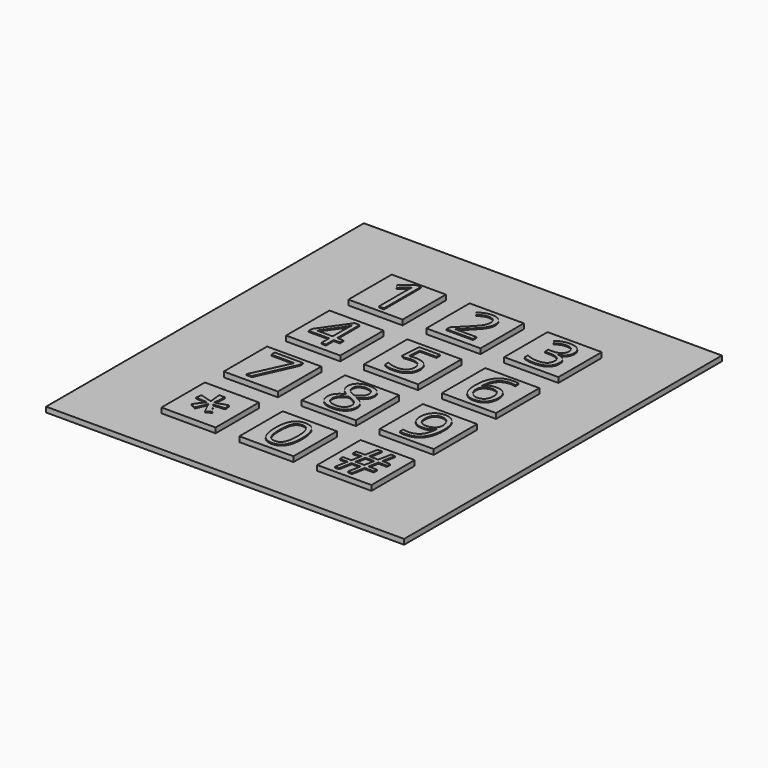
from build123d import *

# Parameters (mm, degrees)
F0_W          = 69.4
F0_H          = 77
F1_DEPTH      = 1
F2_W          = 10.5
F2_H          = 10.5
F3_DEPTH      = 1
F4_TEXT_SIZE  = 12.5769603377
F5_DEPTH      = 0.2
F6_TEXT_SIZE  = 10.9555691274
F7_DEPTH      = 0.2
F8_TEXT_SIZE  = 11.2838111818
F9_DEPTH      = 0.2
F10_TEXT_SIZE = 11.3837614966
F11_DEPTH     = 0.2
F12_TEXT_SIZE = 11.2749830199
F13_DEPTH     = 0.2
F14_TEXT_SIZE = 11.5817846058
F15_DEPTH     = 0.2
F16_TEXT_SIZE = 11.4701903491
F17_DEPTH     = 0.2
F18_TEXT_SIZE = 12.1953906071
F19_DEPTH     = 0.2
F20_TEXT_SIZE = 11.7383821547
F21_DEPTH     = 0.2
F22_TEXT_SIZE = 12.2029864643
F23_DEPTH     = 0.2
F24_TEXT_SIZE = 11.2225185148
F25_DEPTH     = 0.2
F26_TEXT_SIZE = 11.7384957977
F27_DEPTH     = 0.2


# Not quite as in the source:
# - Text() gives the source's letters only with a copy of the font that has no kerning and outlines rounded to 1/6400 em; it was checked with that copy


with BuildPart() as f1:
    # F0 (on Top) → F1 (new body)
    with BuildSketch(Plane.XY):
        with Locations((0.4417933524, 4.7462261665)):
            Rectangle(F0_W, F0_H)
    extrude(amount=F1_DEPTH)


with BuildPart() as f3:
    # F2 (on face) → F3 (new body)
    with BuildSketch(Plane.XY.offset(1)):
        with Locations((-14.0082066476, 25.9962261665)):
            Rectangle(F2_W, F2_H)
    extrude(amount=F3_DEPTH)

    # F4 (on face) → F5 (join)
    with BuildSketch(Plane.XY.offset(2)):
        with Locations((-17.4194090068, 21.5824004263)):
            Text('1', F4_TEXT_SIZE, font='Open Sans', text_align=(TextAlign.LEFT, TextAlign.BOTTOM))
    extrude(amount=F5_DEPTH)


with BuildPart() as f3b:
    # F2 (on face) → F3, piece 2 (new body)
    with BuildSketch(Plane.XY.offset(1)):
        with Locations((-14.0082066476, 10.8962261665)):
            Rectangle(F2_W, F2_H)
    extrude(amount=F3_DEPTH)

    # F10 (on face) → F11 (join)
    with BuildSketch(Plane.XY.offset(2)):
        with Locations((-17.547939904, 6.8340590224)):
            Text('4', F10_TEXT_SIZE, font='Open Sans', text_align=(TextAlign.LEFT, TextAlign.BOTTOM))
    extrude(amount=F11_DEPTH)


with BuildPart() as f3c:
    # F2 (on face) → F3, piece 3 (new body)
    with BuildSketch(Plane.XY.offset(1)):
        with Locations((-14.0082066476, -4.2037738335)):
            Rectangle(F2_W, F2_H)
    extrude(amount=F3_DEPTH)

    # F16 (on face) → F17 (join)
    with BuildSketch(Plane.XY.offset(2)):
        with Locations((-17.3947949011, -8.2585370513)):
            Text('7', F16_TEXT_SIZE, font='Open Sans', text_align=(TextAlign.LEFT, TextAlign.BOTTOM))
    extrude(amount=F17_DEPTH)


with BuildPart() as f3d:
    # F2 (on face) → F3, piece 4 (new body)
    with BuildSketch(Plane.XY.offset(1)):
        with Locations((-14.0082066476, -19.3037738335)):
            Rectangle(F2_W, F2_H)
    extrude(amount=F3_DEPTH)

    # F22 (on face) → F23 (join)
    with BuildSketch(Plane.XY.offset(2)):
        with Locations((-17.4761302769, -25.5072303116)):
            Text('*', F22_TEXT_SIZE, font='Open Sans', text_align=(TextAlign.LEFT, TextAlign.BOTTOM))
    extrude(amount=F23_DEPTH)


with BuildPart() as f3e:
    # F2 (on face) → F3, piece 5 (new body)
    with BuildSketch(Plane.XY.offset(1)):
        with Locations((1.0917933524, 25.9962261665)):
            Rectangle(F2_W, F2_H)
    extrude(amount=F3_DEPTH)

    # F6 (on face) → F7 (join)
    with BuildSketch(Plane.XY.offset(2)):
        with Locations((-1.9074119627, 22.1503581852)):
            Text('2', F6_TEXT_SIZE, font='Open Sans', text_align=(TextAlign.LEFT, TextAlign.BOTTOM))
    extrude(amount=F7_DEPTH)


with BuildPart() as f3f:
    # F2 (on face) → F3, piece 6 (new body)
    with BuildSketch(Plane.XY.offset(1)):
        with Locations((1.0917933524, 10.8962261665)):
            Rectangle(F2_W, F2_H)
    extrude(amount=F3_DEPTH)

    # F12 (on face) → F13 (join)
    with BuildSketch(Plane.XY.offset(2)):
        with Locations((-2.1198638715, 6.924258545)):
            Text('5', F12_TEXT_SIZE, font='Open Sans', text_align=(TextAlign.LEFT, TextAlign.BOTTOM))
    extrude(amount=F13_DEPTH)


with BuildPart() as f3g:
    # F2 (on face) → F3, piece 7 (new body)
    with BuildSketch(Plane.XY.offset(1)):
        with Locations((1.0917933524, -4.2037738335)):
            Rectangle(F2_W, F2_H)
    extrude(amount=F3_DEPTH)

    # F18 (on face) → F19 (join)
    with BuildSketch(Plane.XY.offset(2)):
        with Locations((-2.3180681746, -8.5064787418)):
            Text('8', F18_TEXT_SIZE, font='Open Sans', text_align=(TextAlign.LEFT, TextAlign.BOTTOM))
    extrude(amount=F19_DEPTH)


with BuildPart() as f3h:
    # F2 (on face) → F3, piece 8 (new body)
    with BuildSketch(Plane.XY.offset(1)):
        with Locations((1.0917933524, -19.3037738335)):
            Rectangle(F2_W, F2_H)
    extrude(amount=F3_DEPTH)

    # F24 (on face) → F25 (join)
    with BuildSketch(Plane.XY.offset(2)):
        with Locations((-1.9701938145, -23.3600642532)):
            Text('0', F24_TEXT_SIZE, font='Open Sans', text_align=(TextAlign.LEFT, TextAlign.BOTTOM))
    extrude(amount=F25_DEPTH)


with BuildPart() as f3i:
    # F2 (on face) → F3, piece 9 (new body)
    with BuildSketch(Plane.XY.offset(1)):
        with Locations((16.1917933524, 25.9962261665)):
            Rectangle(F2_W, F2_H)
    extrude(amount=F3_DEPTH)

    # F8 (on face) → F9 (join)
    with BuildSketch(Plane.XY.offset(2)):
        with Locations((13.1029766053, 21.9483301044)):
            Text('3', F8_TEXT_SIZE, font='Open Sans', text_align=(TextAlign.LEFT, TextAlign.BOTTOM))
    extrude(amount=F9_DEPTH)


with BuildPart() as f3j:
    # F2 (on face) → F3, piece 10 (new body)
    with BuildSketch(Plane.XY.offset(1)):
        with Locations((16.1917933524, 10.8962261665)):
            Rectangle(F2_W, F2_H)
    extrude(amount=F3_DEPTH)

    # F14 (on face) → F15 (join)
    with BuildSketch(Plane.XY.offset(2)):
        with Locations((12.8183374181, 6.8138097413)):
            Text('6', F14_TEXT_SIZE, font='Open Sans', text_align=(TextAlign.LEFT, TextAlign.BOTTOM))
    extrude(amount=F15_DEPTH)


with BuildPart() as f3k:
    # F2 (on face) → F3, piece 11 (new body)
    with BuildSketch(Plane.XY.offset(1)):
        with Locations((16.1917933524, -4.2037738335)):
            Rectangle(F2_W, F2_H)
    extrude(amount=F3_DEPTH)

    # F20 (on face) → F21 (join)
    with BuildSketch(Plane.XY.offset(2)):
        with Locations((12.8407233631, -8.4516351514)):
            Text('9', F20_TEXT_SIZE, font='Open Sans', text_align=(TextAlign.LEFT, TextAlign.BOTTOM))
    extrude(amount=F21_DEPTH)


with BuildPart() as f3l:
    # F2 (on face) → F3, piece 12 (new body)
    with BuildSketch(Plane.XY.offset(1)):
        with Locations((16.1917933524, -19.3037738335)):
            Rectangle(F2_W, F2_H)
    extrude(amount=F3_DEPTH)

    # F26 (on face) → F27 (join)
    with BuildSketch(Plane.XY.offset(2)):
        with Locations((12.2862746939, -23.5922522843)):
            Text('#', F26_TEXT_SIZE, font='Open Sans', text_align=(TextAlign.LEFT, TextAlign.BOTTOM))
    extrude(amount=F27_DEPTH)


solid = Compound([f1.part, f3.part, f3b.part, f3c.part, f3d.part, f3e.part, f3f.part, f3g.part, f3h.part, f3i.part, f3j.part, f3k.part, f3l.part])
